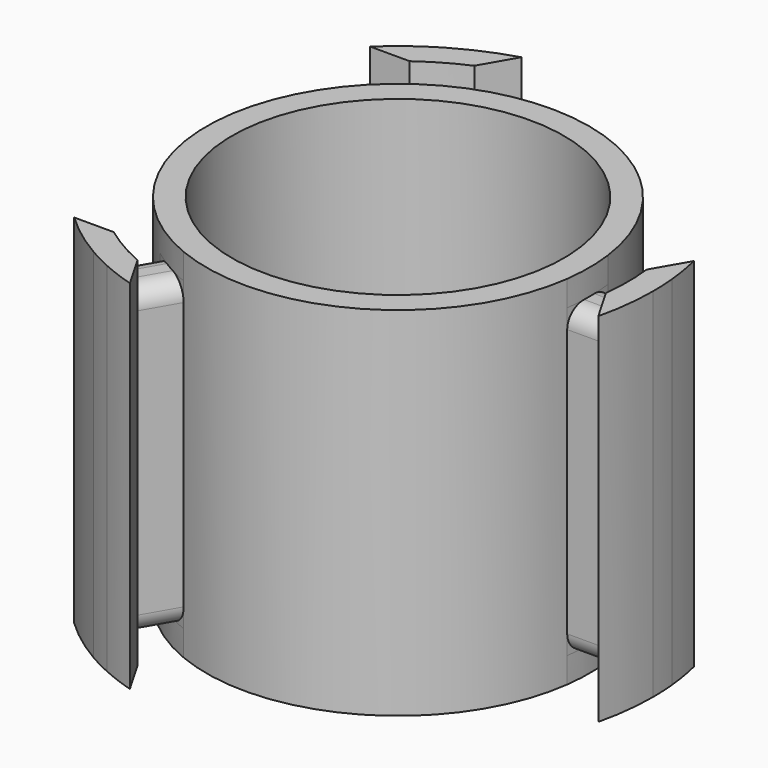
from build123d import *

# Parameters (mm, degrees)
F1_DEPTH     = 28
F2_R         = 18
F2_R_2       = 15
F3_DEPTH     = 2
F4_R         = 18.0111355842
F4_R_2       = 15
F5_DEPTH     = 2
F6_T4_DEPTH  = 10.5336799948
F6_S5_R      = 15
F6_T6_DEPTH  = 7
F6_S7_R      = 18.0111355842
F6_T8_DEPTH  = 7
F6_T12_DEPTH = 10.5336799948
F6_S13_R     = 15
F6_T14_DEPTH = 7
F6_S15_R     = 18.0111355842
F6_T16_DEPTH = 7
F6_T20_DEPTH = 10.5336799948
F6_S21_R     = 15
F6_T22_DEPTH = 7
F6_S23_R     = 18.0111355842
F6_T24_DEPTH = 7
F6_T28_DEPTH = 10.5336799948
F6_S29_R     = 15
F6_T30_DEPTH = 7
F6_S31_R     = 18.0111355842
F6_T32_DEPTH = 7
F6_T36_DEPTH = 10.5336799948
F6_S37_R     = 15
F6_T38_DEPTH = 7
F6_S39_R     = 18.0111355842
F6_T40_DEPTH = 7
F6_T44_DEPTH = 10.5336799948
F6_S45_R     = 15
F6_T46_DEPTH = 7
F6_S47_R     = 18.0111355842
F6_T48_DEPTH = 7
F6_T52_DEPTH = 10.5224750727
F6_S53_R     = 15
F6_T54_DEPTH = 7
F6_S55_R     = 18
F6_T56_DEPTH = 7
F6_T60_DEPTH = 10.5224750727
F6_S61_R     = 15
F6_T62_DEPTH = 7
F6_S63_R     = 18
F6_T64_DEPTH = 7
F6_T68_DEPTH = 10.5224750727
F6_S69_R     = 15
F6_T70_DEPTH = 7
F6_S71_R     = 18
F6_T72_DEPTH = 7
F6_T76_DEPTH = 10.5224750727
F6_S77_R     = 15
F6_T78_DEPTH = 7
F6_S79_R     = 18
F6_T80_DEPTH = 7
F6_T84_DEPTH = 10.5224750727
F6_S85_R     = 15
F6_T86_DEPTH = 7
F6_S87_R     = 18
F6_T88_DEPTH = 7
F6_T92_DEPTH = 10.5224750727
F6_S93_R     = 15
F6_T94_DEPTH = 7
F6_S95_R     = 18
F6_T96_DEPTH = 7


# Not quite as in the source:
# - a fillet or chamfer that OpenCascade refuses, or shapes differently, is made with other operations: its cross-section is extruded or revolved along the edge and cut away or added


with BuildPart() as f1:
    # F0 (on Top) → F1 (new body)
    with BuildSketch(Plane.XY):
        with BuildLine():
            Line((15, 0), (13, 0))
            ThreePointArc((13, 0), (6.5, -11.2583302492), (-6.5, -11.2583302492))
            Line((-6.5, -11.2583302492), (-7.5, -12.9903810568))
            ThreePointArc((-7.5, -12.9903810568), (-6.6152748349, -13.4624714989), (-5.7009835661, -13.8743931896))
            ThreePointArc((-5.7009835661, -13.8743931896), (7.5, -12.9903810568), (14.8660687473, -2))
            ThreePointArc((14.8660687473, -2), (14.9664797332, -1.0022396895), (15, 0))
        make_face()
        with BuildLine():
            ThreePointArc((-6.5, 11.2583302492), (6.5, 11.2583302492), (13, 0))
            Line((13, 0), (15, 0))
            ThreePointArc((15, 0), (14.9664797332, 1.0022396895), (14.8660687473, 2))
            ThreePointArc((14.8660687473, 2), (7.5, 12.9903810568), (-5.7009835661, 13.8743931896))
            ThreePointArc((-5.7009835661, 13.8743931896), (-6.6152748349, 13.4624714989), (-7.5, 12.9903810568))
            Line((-7.5, 12.9903810568), (-6.5, 11.2583302492))
        make_face()
        with BuildLine():
            ThreePointArc((-6.5, -11.2583302492), (-13, 0), (-6.5, 11.2583302492))
            Line((-6.5, 11.2583302492), (-7.5, 12.9903810568))
            ThreePointArc((-7.5, 12.9903810568), (-8.3512048984, 12.4602318095), (-9.1650851812, 11.8743931896))
            ThreePointArc((-9.1650851812, 11.8743931896), (-15, 0), (-9.1650851812, -11.8743931896))
            ThreePointArc((-9.1650851812, -11.8743931896), (-8.3512048984, -12.4602318095), (-7.5, -12.9903810568))
            Line((-7.5, -12.9903810568), (-6.5, -11.2583302492))
        make_face()
        with BuildLine():
            Line((20, 0), (15, 0))
            ThreePointArc((15, 0), (14.9664797332, -1.0022396895), (14.8660687473, -2))
            Line((14.8660687473, -2), (17.8997487421, -2))
            Line((17.8997487421, -2), (19.4454130574, -4.6771691254))
            ThreePointArc((19.4454130574, -4.6771691254), (19.8608693308, -2.3549669692), (20, 0))
        make_face()
        with BuildLine():
            ThreePointArc((14.8660687473, 2), (14.9664797332, 1.0022396895), (15, 0))
            Line((15, 0), (20, 0))
            ThreePointArc((20, 0), (19.9749214622, 1.0012555012), (19.8997487421, 2))
            Line((19.8997487421, 2), (17.8997487421, 2))
            Line((17.8997487421, 2), (14.8660687473, 2))
        make_face()
        with BuildLine():
            Line((-10, 17.3205080757), (-7.5, 12.9903810568))
            ThreePointArc((-7.5, 12.9903810568), (-6.6152748349, 13.4624714989), (-5.7009835661, 13.8743931896))
            Line((-5.7009835661, 13.8743931896), (-7.2178235635, 16.501637132))
            Line((-7.2178235635, 16.501637132), (-5.6721592483, 19.1788062575))
            ThreePointArc((-5.6721592483, 19.1788062575), (-7.8909734449, 18.3775008663), (-10, 17.3205080757))
        make_face()
        with BuildLine():
            ThreePointArc((-9.1650851812, 11.8743931896), (-8.3512048984, 12.4602318095), (-7.5, 12.9903810568))
            Line((-7.5, 12.9903810568), (-10, 17.3205080757))
            ThreePointArc((-10, 17.3205080757), (-10.8545734308, 16.7981616743), (-11.6819251786, 16.2336879396))
            Line((-11.6819251786, 16.2336879396), (-10.6819251786, 14.501637132))
            Line((-10.6819251786, 14.501637132), (-9.1650851812, 11.8743931896))
        make_face()
        with BuildLine():
            Line((-10, -17.3205080757), (-7.5, -12.9903810568))
            ThreePointArc((-7.5, -12.9903810568), (-8.3512048984, -12.4602318095), (-9.1650851812, -11.8743931896))
            Line((-9.1650851812, -11.8743931896), (-10.6819251786, -14.501637132))
            Line((-10.6819251786, -14.501637132), (-13.7732538091, -14.501637132))
            ThreePointArc((-13.7732538091, -14.501637132), (-11.9698958858, -16.0225338971), (-10, -17.3205080757))
        make_face()
        with BuildLine():
            ThreePointArc((-5.7009835661, -13.8743931896), (-6.6152748349, -13.4624714989), (-7.5, -12.9903810568))
            Line((-7.5, -12.9903810568), (-10, -17.3205080757))
            ThreePointArc((-10, -17.3205080757), (-9.1203480314, -17.7994171755), (-8.2178235635, -18.2336879396))
            Line((-8.2178235635, -18.2336879396), (-7.2178235635, -16.501637132))
            Line((-7.2178235635, -16.501637132), (-5.7009835661, -13.8743931896))
        make_face()
        with BuildLine():
            Line((19.4454130574, 4.6771691254), (17.8997487421, 2))
            Line((17.8997487421, 2), (19.8997487421, 2))
            ThreePointArc((19.8997487421, 2), (19.718069071, 3.3463042466), (19.4454130574, 4.6771691254))
        make_face()
        with BuildLine():
            Line((-13.7732538091, 14.501637132), (-10.6819251786, 14.501637132))
            Line((-10.6819251786, 14.501637132), (-11.6819251786, 16.2336879396))
            ThreePointArc((-11.6819251786, 16.2336879396), (-12.7570190219, 15.4031966057), (-13.7732538091, 14.501637132))
        make_face()
        with BuildLine():
            Line((-5.6721592483, -19.1788062575), (-7.2178235635, -16.501637132))
            Line((-7.2178235635, -16.501637132), (-8.2178235635, -18.2336879396))
            ThreePointArc((-8.2178235635, -18.2336879396), (-6.9610500491, -18.7495008524), (-5.6721592483, -19.1788062575))
        make_face()
    extrude(amount=F1_DEPTH)

    # F2 (on Top) → F3 (cut)
    with BuildSketch(Plane.XY):
        Circle(F2_R)
        Circle(F2_R_2, mode=Mode.SUBTRACT)
    extrude(amount=F3_DEPTH, mode=Mode.SUBTRACT)

    # F4 (on face) → F5 (cut)
    with BuildSketch(Plane.XY.offset(28)):
        Circle(F4_R)
        Circle(F4_R_2, mode=Mode.SUBTRACT)
    extrude(amount=-F5_DEPTH, mode=Mode.SUBTRACT)

    # F6: fillet of radius 1.5 on 12 edges, made by hand


with BuildPart() as f6_tool2:
    # F6_s3 → F6_t4 (new body)
    with BuildSketch(Plane(origin=(-10.8248743711, -18.7492323962, 0), x_dir=(0, 0, 1), z_dir=(0.5, 0.8660254038, 0))):
        with BuildLine():
            ThreePointArc((26, 0.5), (25.5606601718, 1.5606601718), (24.5, 2))
            Line((24.5, 2), (26, 2))
            Line((26, 2), (26, 0.5))
        make_face()
    extrude(amount=F6_T4_DEPTH)

    # F6_s5 → F6_t6 (cut, symmetric)
    with BuildSketch(Plane.XY.offset(25.2)):
        Circle(F6_S5_R)
    extrude(amount=F6_T6_DEPTH, both=True, mode=Mode.SUBTRACT)

    # F6_s7 → F6_t8 (intersect, symmetric)
    with BuildSketch(Plane.XY.offset(25.2)):
        Circle(F6_S7_R)
    extrude(amount=F6_T8_DEPTH, both=True, mode=Mode.INTERSECT)


with BuildPart() as f1_1:
    add(f1.part)

    # F6_t1: cut F6_tool2
    add(f6_tool2.part, mode=Mode.SUBTRACT)


with BuildPart() as f6_tool10:
    # F6_s11 → F6_t12 (new body)
    with BuildSketch(Plane(origin=(-5.5580343737, -9.6267979254, 0), x_dir=(0, 0, 1), z_dir=(-0.5, -0.8660254038, 0))):
        with BuildLine():
            ThreePointArc((24.5, 2), (25.5606601718, 1.5606601718), (26, 0.5))
            Line((26, 0.5), (26, 2))
            Line((26, 2), (24.5, 2))
        make_face()
    extrude(amount=F6_T12_DEPTH)

    # F6_s13 → F6_t14 (cut, symmetric)
    with BuildSketch(Plane.XY.offset(25.2)):
        Circle(F6_S13_R)
    extrude(amount=F6_T14_DEPTH, both=True, mode=Mode.SUBTRACT)

    # F6_s15 → F6_t16 (intersect, symmetric)
    with BuildSketch(Plane.XY.offset(25.2)):
        Circle(F6_S15_R)
    extrude(amount=F6_T16_DEPTH, both=True, mode=Mode.INTERSECT)


with BuildPart() as f1_2:
    add(f1_1.part)

    # F6_t9: cut F6_tool10
    add(f6_tool10.part, mode=Mode.SUBTRACT)


with BuildPart() as f6_tool18:
    # F6_s19 → F6_t20 (new body)
    with BuildSketch(Plane.YZ.offset(11.1160687473)):
        with BuildLine():
            ThreePointArc((-2, 24.5), (-1.5606601718, 25.5606601718), (-0.5, 26))
            Line((-0.5, 26), (-2, 26))
            Line((-2, 26), (-2, 24.5))
        make_face()
    extrude(amount=F6_T20_DEPTH)

    # F6_s21 → F6_t22 (cut, symmetric)
    with BuildSketch(Plane.XY.offset(25.2)):
        Circle(F6_S21_R)
    extrude(amount=F6_T22_DEPTH, both=True, mode=Mode.SUBTRACT)

    # F6_s23 → F6_t24 (intersect, symmetric)
    with BuildSketch(Plane.XY.offset(25.2)):
        Circle(F6_S23_R)
    extrude(amount=F6_T24_DEPTH, both=True, mode=Mode.INTERSECT)


with BuildPart() as f1_3:
    add(f1_2.part)

    # F6_t17: cut F6_tool18
    add(f6_tool18.part, mode=Mode.SUBTRACT)


with BuildPart() as f6_tool26:
    # F6_s27 → F6_t28 (new body)
    with BuildSketch(Plane.YZ.offset(21.6497487421)):
        with BuildLine():
            ThreePointArc((2, 24.5), (1.5606601718, 25.5606601718), (0.5, 26))
            Line((0.5, 26), (2, 26))
            Line((2, 26), (2, 24.5))
        make_face()
    extrude(amount=-F6_T28_DEPTH)

    # F6_s29 → F6_t30 (cut, symmetric)
    with BuildSketch(Plane.XY.offset(25.2)):
        Circle(F6_S29_R)
    extrude(amount=F6_T30_DEPTH, both=True, mode=Mode.SUBTRACT)

    # F6_s31 → F6_t32 (intersect, symmetric)
    with BuildSketch(Plane.XY.offset(25.2)):
        Circle(F6_S31_R)
    extrude(amount=F6_T32_DEPTH, both=True, mode=Mode.INTERSECT)


with BuildPart() as f1_4:
    add(f1_3.part)

    # F6_t25: cut F6_tool26
    add(f6_tool26.part, mode=Mode.SUBTRACT)


with BuildPart() as f6_tool34:
    # F6_s35 → F6_t36 (new body)
    with BuildSketch(Plane(origin=(-5.5580343737, 9.6267979254, 0), x_dir=(0, 0, 1), z_dir=(-0.5, 0.8660254038, 0))):
        with BuildLine():
            ThreePointArc((24.5, 2), (25.5606601718, 1.5606601718), (26, 0.5))
            Line((26, 0.5), (26, 2))
            Line((26, 2), (24.5, 2))
        make_face()
    extrude(amount=F6_T36_DEPTH)

    # F6_s37 → F6_t38 (cut, symmetric)
    with BuildSketch(Plane.XY.offset(25.2)):
        Circle(F6_S37_R)
    extrude(amount=F6_T38_DEPTH, both=True, mode=Mode.SUBTRACT)

    # F6_s39 → F6_t40 (intersect, symmetric)
    with BuildSketch(Plane.XY.offset(25.2)):
        Circle(F6_S39_R)
    extrude(amount=F6_T40_DEPTH, both=True, mode=Mode.INTERSECT)


with BuildPart() as f1_5:
    add(f1_4.part)

    # F6_t33: cut F6_tool34
    add(f6_tool34.part, mode=Mode.SUBTRACT)


with BuildPart() as f6_tool42:
    # F6_s43 → F6_t44 (new body)
    with BuildSketch(Plane(origin=(-10.8248743711, 18.7492323962, 0), x_dir=(0, 0, 1), z_dir=(0.5, -0.8660254038, 0))):
        with BuildLine():
            ThreePointArc((26, 0.5), (25.5606601718, 1.5606601718), (24.5, 2))
            Line((24.5, 2), (26, 2))
            Line((26, 2), (26, 0.5))
        make_face()
    extrude(amount=F6_T44_DEPTH)

    # F6_s45 → F6_t46 (cut, symmetric)
    with BuildSketch(Plane.XY.offset(25.3)):
        Circle(F6_S45_R)
    extrude(amount=F6_T46_DEPTH, both=True, mode=Mode.SUBTRACT)

    # F6_s47 → F6_t48 (intersect, symmetric)
    with BuildSketch(Plane.XY.offset(25.3)):
        Circle(F6_S47_R)
    extrude(amount=F6_T48_DEPTH, both=True, mode=Mode.INTERSECT)


with BuildPart() as f1_6:
    add(f1_5.part)

    # F6_t41: cut F6_tool42
    add(f6_tool42.part, mode=Mode.SUBTRACT)


with BuildPart() as f6_tool50:
    # F6_s51 → F6_t52 (new body)
    with BuildSketch(Plane(origin=(-10.81927191, 18.739528649, 0), x_dir=(0, 0, 1), z_dir=(0.5, -0.8660254038, 0))):
        with BuildLine():
            ThreePointArc((2, 0.5), (2.4393398282, 1.5606601718), (3.5, 2))
            Line((3.5, 2), (2, 2))
            Line((2, 2), (2, 0.5))
        make_face()
    extrude(amount=F6_T52_DEPTH)

    # F6_s53 → F6_t54 (cut, symmetric)
    with BuildSketch(Plane.XY.offset(2.8)):
        Circle(F6_S53_R)
    extrude(amount=F6_T54_DEPTH, both=True, mode=Mode.SUBTRACT)

    # F6_s55 → F6_t56 (intersect, symmetric)
    with BuildSketch(Plane.XY.offset(2.8)):
        Circle(F6_S55_R)
    extrude(amount=F6_T56_DEPTH, both=True, mode=Mode.INTERSECT)


with BuildPart() as f1_7:
    add(f1_6.part)

    # F6_t49: cut F6_tool50
    add(f6_tool50.part, mode=Mode.SUBTRACT)


with BuildPart() as f6_tool58:
    # F6_s59 → F6_t60 (new body)
    with BuildSketch(Plane(origin=(-5.5580343737, 9.6267979254, 0), x_dir=(0, 0, 1), z_dir=(-0.5, 0.8660254038, 0))):
        with BuildLine():
            ThreePointArc((2, 0.5), (2.4393398282, 1.5606601718), (3.5, 2))
            Line((3.5, 2), (2, 2))
            Line((2, 2), (2, 0.5))
        make_face()
    extrude(amount=F6_T60_DEPTH)

    # F6_s61 → F6_t62 (cut, symmetric)
    with BuildSketch(Plane.XY.offset(2.8)):
        Circle(F6_S61_R)
    extrude(amount=F6_T62_DEPTH, both=True, mode=Mode.SUBTRACT)

    # F6_s63 → F6_t64 (intersect, symmetric)
    with BuildSketch(Plane.XY.offset(2.8)):
        Circle(F6_S63_R)
    extrude(amount=F6_T64_DEPTH, both=True, mode=Mode.INTERSECT)


with BuildPart() as f1_8:
    add(f1_7.part)

    # F6_t57: cut F6_tool58
    add(f6_tool58.part, mode=Mode.SUBTRACT)


with BuildPart() as f6_tool66:
    # F6_s67 → F6_t68 (new body)
    with BuildSketch(Plane.YZ.offset(21.63854382)):
        with BuildLine():
            ThreePointArc((2, 3.5), (1.5606601718, 2.4393398282), (0.5, 2))
            Line((0.5, 2), (2, 2))
            Line((2, 2), (2, 3.5))
        make_face()
    extrude(amount=-F6_T68_DEPTH)

    # F6_s69 → F6_t70 (cut, symmetric)
    with BuildSketch(Plane.XY.offset(2.8)):
        Circle(F6_S69_R)
    extrude(amount=F6_T70_DEPTH, both=True, mode=Mode.SUBTRACT)

    # F6_s71 → F6_t72 (intersect, symmetric)
    with BuildSketch(Plane.XY.offset(2.8)):
        Circle(F6_S71_R)
    extrude(amount=F6_T72_DEPTH, both=True, mode=Mode.INTERSECT)


with BuildPart() as f1_9:
    add(f1_8.part)

    # F6_t65: cut F6_tool66
    add(f6_tool66.part, mode=Mode.SUBTRACT)


with BuildPart() as f6_tool74:
    # F6_s75 → F6_t76 (new body)
    with BuildSketch(Plane.YZ.offset(11.1160687473)):
        with BuildLine():
            ThreePointArc((-2, 3.5), (-1.5606601718, 2.4393398282), (-0.5, 2))
            Line((-0.5, 2), (-2, 2))
            Line((-2, 2), (-2, 3.5))
        make_face()
    extrude(amount=F6_T76_DEPTH)

    # F6_s77 → F6_t78 (cut, symmetric)
    with BuildSketch(Plane.XY.offset(2.8)):
        Circle(F6_S77_R)
    extrude(amount=F6_T78_DEPTH, both=True, mode=Mode.SUBTRACT)

    # F6_s79 → F6_t80 (intersect, symmetric)
    with BuildSketch(Plane.XY.offset(2.8)):
        Circle(F6_S79_R)
    extrude(amount=F6_T80_DEPTH, both=True, mode=Mode.INTERSECT)


with BuildPart() as f1_10:
    add(f1_9.part)

    # F6_t73: cut F6_tool74
    add(f6_tool74.part, mode=Mode.SUBTRACT)


with BuildPart() as f6_tool82:
    # F6_s83 → F6_t84 (new body)
    with BuildSketch(Plane(origin=(-5.5580343737, -9.6267979254, 0), x_dir=(0, 0, 1), z_dir=(-0.5, -0.8660254038, 0))):
        with BuildLine():
            ThreePointArc((2, 0.5), (2.4393398282, 1.5606601718), (3.5, 2))
            Line((3.5, 2), (2, 2))
            Line((2, 2), (2, 0.5))
        make_face()
    extrude(amount=F6_T84_DEPTH)

    # F6_s85 → F6_t86 (cut, symmetric)
    with BuildSketch(Plane.XY.offset(2.8)):
        Circle(F6_S85_R)
    extrude(amount=F6_T86_DEPTH, both=True, mode=Mode.SUBTRACT)

    # F6_s87 → F6_t88 (intersect, symmetric)
    with BuildSketch(Plane.XY.offset(2.8)):
        Circle(F6_S87_R)
    extrude(amount=F6_T88_DEPTH, both=True, mode=Mode.INTERSECT)


with BuildPart() as f1_11:
    add(f1_10.part)

    # F6_t81: cut F6_tool82
    add(f6_tool82.part, mode=Mode.SUBTRACT)


with BuildPart() as f6_tool90:
    # F6_s91 → F6_t92 (new body)
    with BuildSketch(Plane(origin=(-10.81927191, -18.739528649, 0), x_dir=(0, 0, 1), z_dir=(0.5, 0.8660254038, 0))):
        with BuildLine():
            ThreePointArc((2, 0.5), (2.4393398282, 1.5606601718), (3.5, 2))
            Line((3.5, 2), (2, 2))
            Line((2, 2), (2, 0.5))
        make_face()
    extrude(amount=F6_T92_DEPTH)

    # F6_s93 → F6_t94 (cut, symmetric)
    with BuildSketch(Plane.XY.offset(2.8)):
        Circle(F6_S93_R)
    extrude(amount=F6_T94_DEPTH, both=True, mode=Mode.SUBTRACT)

    # F6_s95 → F6_t96 (intersect, symmetric)
    with BuildSketch(Plane.XY.offset(2.8)):
        Circle(F6_S95_R)
    extrude(amount=F6_T96_DEPTH, both=True, mode=Mode.INTERSECT)


with BuildPart() as f1_12:
    add(f1_11.part)

    # F6_t89: cut F6_tool90
    add(f6_tool90.part, mode=Mode.SUBTRACT)


solid = f1_12.part
